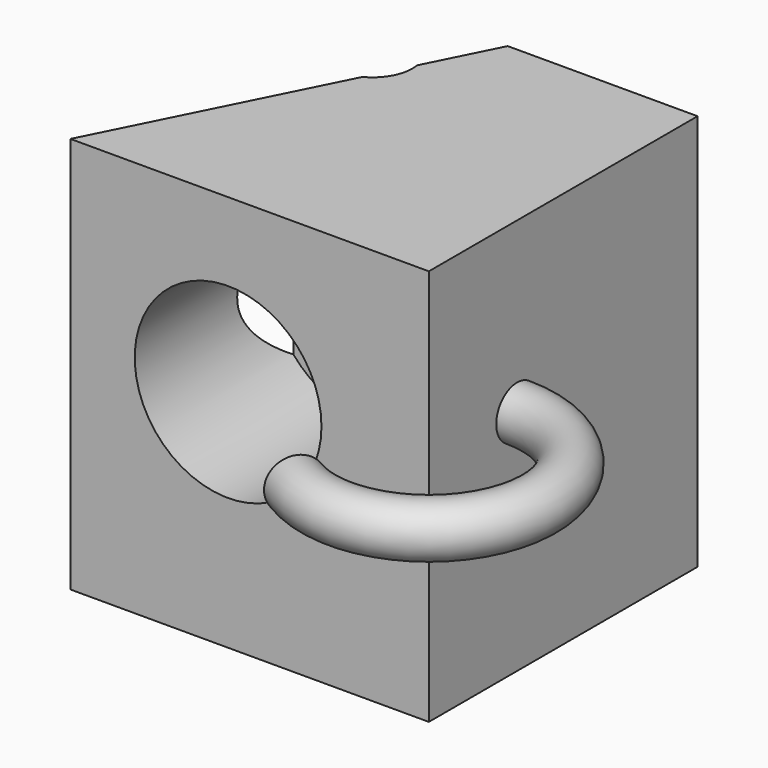
from build123d import *

# Parameters (mm, degrees)
F1_DEPTH = 30
F2_R     = 7.0607743661
F3_DEPTH = 12.95017
F4_R     = 1.9790251597
F5_ANGLE = 211.8266616901


# Not quite as in the source:
# - a feature of the source that left no trace in its solid (it failed there, or was rolled back) is left out


with BuildPart() as f1:
    # F0 (on Top) → F1 (new body)
    with BuildSketch(Plane.XY):
        with BuildLine():
            Line((-8.5449986998, 1.5012763055), (-22.9009841796, 1.5012763055))
            Line((-22.9009841796, 1.5012763055), (-25.5437633875, -3.7646328319))
            ThreePointArc((-25.5437633875, -3.7646328319), (-25.5119398754, -4.015202253), (-25.5013069136, -4.2675605514))
            ThreePointArc((-25.5013069136, -4.2675605514), (-25.9427272038, -5.8339799934), (-27.1370868258, -6.9394332191))
            Line((-27.1370868258, -6.9394332191), (-35.6483731166, -23.8987236945))
            Line((-35.6483731166, -23.8987236945), (-8.5449986998, -23.8987236945))
            Line((-8.5449986998, -23.8987236945), (-8.5449986998, 1.5012763055))
        make_face()
    extrude(amount=F1_DEPTH)

    # F2 (on face) → F3 (cut)
    with BuildSketch(Plane.XZ.offset(23.8987236945)):
        with Locations((-23.7271394581, 17.0257668942)):
            Circle(F2_R)
    extrude(amount=-F3_DEPTH, mode=Mode.SUBTRACT)

    # F4 (on face) → F5 (revolve)
    with BuildSketch(Plane.YZ.offset(-8.5449986998)):
        with Locations((-15.5504914001, 17.2328893095)):
            Circle(F4_R)
    revolve(axis=Axis((-8.5449986998, -23.8987236945, 15), (0, 0, -1)), revolution_arc=F5_ANGLE)


solid = f1.part
